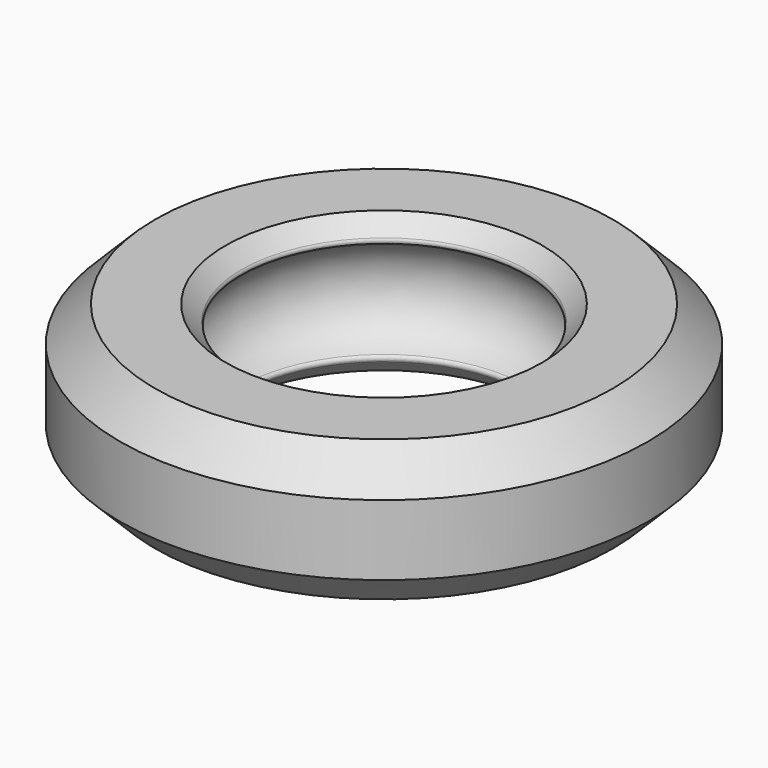
from build123d import *

# Parameters (mm, degrees)
F3_R = 1


# Not quite as in the source:
# - a fillet or chamfer that OpenCascade refuses, or shapes differently, is made with other operations: its cross-section is extruded or revolved along the edge and cut away or added


with BuildPart() as f1:
    # F0 (on Front) → F1 (revolve)
    with BuildSketch(Plane.XZ):
        with BuildLine():
            Line((0, 5), (0, 0))
            Line((0, 0), (40, 0))
            Line((40, 0), (40, 40))
            Line((40, 40), (0, 40))
            Line((0, 40), (0, 35))
            ThreePointArc((0, 35), (15, 20), (0, 5))
        make_face()
    revolve(axis=Axis((-35, 0, 22.5124461576), (0, 0, -1)))

    # F2: chamfer of 10 on 4 edges, made by hand

    # F2_s1 → F2_t2 (revolve, cut)
    with BuildSketch(Plane.XZ):
        Polygon((30, 0), (40, 10), (40, 0), align=None)
    revolve(axis=Axis((-35, 0, 0), (0, 0, -1)), mode=Mode.SUBTRACT)

    # F2_s3 → F2_t4 (revolve, cut)
    with BuildSketch(Plane.XZ):
        Polygon((40, 30), (30, 40), (40, 40), align=None)
    revolve(axis=Axis((-35, 0, 40), (0, 0, -1)), mode=Mode.SUBTRACT)

    # F2_s5 → F2_t6 (revolve, cut)
    with BuildSketch(Plane.XZ):
        Polygon((0, 10), (10, 0), (0, 0), align=None)
    revolve(axis=Axis((-35, 0, 0), (0, 0, -1)), mode=Mode.SUBTRACT)

    # F2_s7 → F2_t8 (revolve, cut)
    with BuildSketch(Plane.XZ):
        Polygon((10, 40), (0, 30), (0, 40), align=None)
    revolve(axis=Axis((-35, 0, 40), (0, 0, -1)), mode=Mode.SUBTRACT)

    # F3
    f3_edges = [f1.edges().sort_by_distance(p)[0] for p in [
        (-74.354143, 0, 34.354143),
        (-74.354143, 0, 5.645857),
    ]]
    fillet(f3_edges, radius=F3_R)


solid = f1.part
